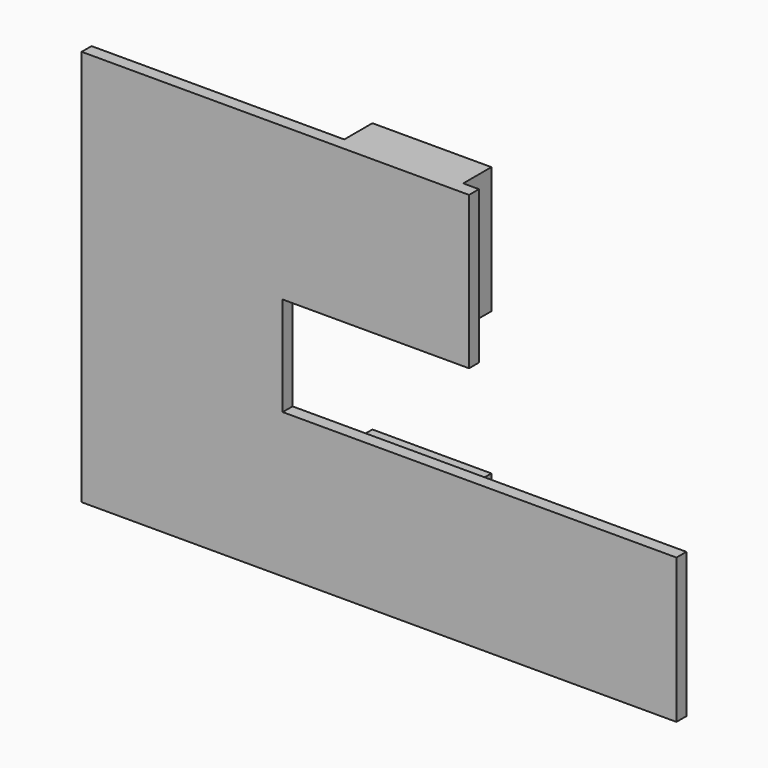
from build123d import *

# Parameters (mm, degrees)
F1_DEPTH = 3.175
F0_W     = 30.48
F0_H     = 32.512
F2_DEPTH = 12.192


with BuildPart() as f1:
    # F0 (on Front) → F1 (new body)
    with BuildSketch(Plane.XZ):
        Polygon((-11.6948662326, 48.9731033504), (-76.444491744, 48.9731033504), (-76.444491744, -52.6268966496), (-11.6948662326, -52.6268966496), (-11.6948662326, -20.1148966496), (18.7851337674, -20.1148966496), (18.7851337674, -52.6268966496), (75.955508256, -52.6268966496), (75.955508256, -15.5456149951), (22.8138189573, -15.5456149951), (-24.9381810427, -15.5456149951), (-24.9381810427, 9.8543850049), (22.8138189573, 9.8543850049), (22.8138189573, 48.9731033504), (18.7851337674, 48.9731033504), (18.7851337674, 16.4611033504), (-11.6948662326, 16.4611033504), align=None)
    extrude(amount=-F1_DEPTH)

    # F0 (on Front) → F2 (join)
    with BuildSketch(Plane.XZ):
        with Locations((3.5451337674, 32.7171033504)):
            Rectangle(F0_W, F0_H)
        with Locations((3.5451337674, -36.3708966496)):
            Rectangle(F0_W, F0_H)
    extrude(amount=-F2_DEPTH)


solid = f1.part
